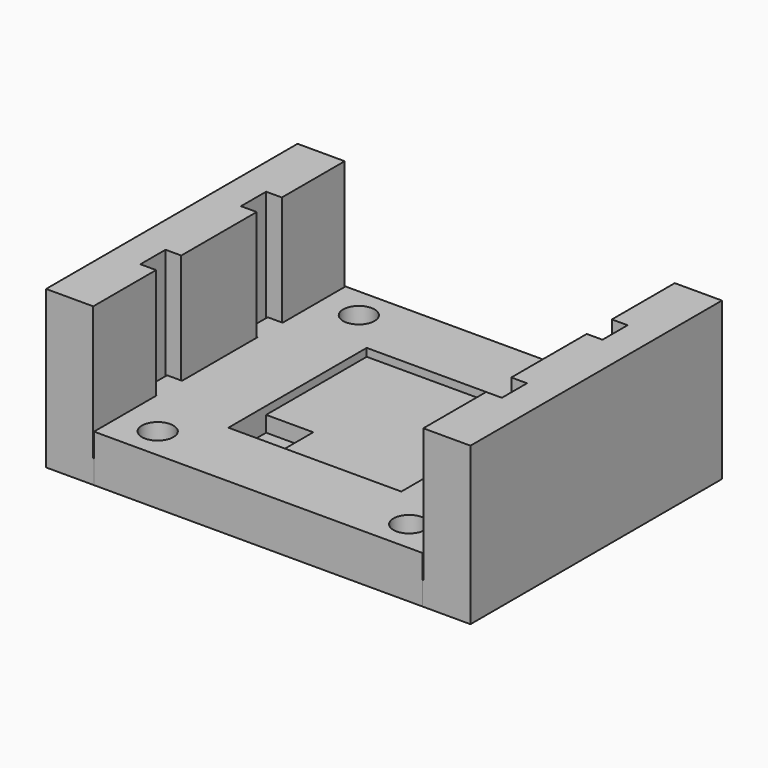
from build123d import *

# Parameters (mm, degrees)
F0_W      = 54
F0_H      = 40
F0_R      = 2
F0_R_2    = 3
F1_DEPTH  = 3
F3_DEPTH  = 20
F4_W      = 41.8
F4_H      = 40
F5_DEPTH  = 6
F7_START  = 5
F6_W      = 22
F6_H      = 22
F7_DEPTH  = 1
F9_START  = 2.5
F8_W      = 6
F8_H      = 6
F9_DEPTH  = 2.5
F12_R     = 2
F13_DEPTH = 25
F14_W     = 2
F14_H     = 4
F15_DEPTH = 6


# Not quite as in the source:
# - a feature of the source that left no trace in its solid (it failed there, or was rolled back) is left out


with BuildPart() as f1:
    # F0 (on Top) → F1 (new body)
    with BuildSketch(Plane.XY):
        Rectangle(F0_W, F0_H)
        with Locations((-16, -16)):
            Circle(F0_R, mode=Mode.SUBTRACT)
        with Locations((-4, -4)):
            Circle(F0_R_2, mode=Mode.SUBTRACT)
        with Locations((16, -16)):
            Circle(F0_R, mode=Mode.SUBTRACT)
        with Locations((4, -4)):
            Circle(F0_R_2, mode=Mode.SUBTRACT)
        with Locations((-4, 4)):
            Circle(F0_R_2, mode=Mode.SUBTRACT)
        with Locations((-16, 16)):
            Circle(F0_R, mode=Mode.SUBTRACT)
        with Locations((4, 4)):
            Circle(F0_R_2, mode=Mode.SUBTRACT)
        with Locations((16, 16)):
            Circle(F0_R, mode=Mode.SUBTRACT)
    extrude(amount=F1_DEPTH)

    # F2 (on Top) → F3 (join)
    with BuildSketch(Plane.XY):
        Polygon((-27, 12.5), (-27, -20), (-21, -20), (-21, -10), (-23, -10), (-23, -6), (-21, -6), (-21, 6), (-23, 6), (-23, 10), (-21, 10), (-21, 20), (-27, 20), align=None)
        Polygon((27, 20), (21, 20), (21, 10), (23, 10), (23, 6), (21, 6), (21, -6), (23, -6), (23, -10), (21, -10), (21, -20), (27, -20), align=None)
    extrude(amount=F3_DEPTH)


with BuildPart() as f5:
    # F4 (on Top) → F5 (new body)
    with BuildSketch(Plane.XY):
        Rectangle(F4_W, F4_H)
    extrude(amount=F5_DEPTH)

    # F6 (on Top) → F7 (cut)
    with BuildSketch(Plane.XY.offset(F7_START)):
        Rectangle(F6_W, F6_H)
    extrude(amount=F7_DEPTH, mode=Mode.SUBTRACT)

    # F8 (on Top) → F9 (cut)
    with BuildSketch(Plane.XY.offset(F9_START)):
        with Locations((-8, -8)):
            Rectangle(F8_W, F8_H)
    extrude(amount=F9_DEPTH, mode=Mode.SUBTRACT)

    # F12 (on Top) → F13 (cut)
    with BuildSketch(Plane.XY):
        with Locations((-16, 16)):
            Circle(F12_R)
        with Locations((16, 16)):
            Circle(F12_R)
        with Locations((16, -16)):
            Circle(F12_R)
        with Locations((-16, -16)):
            Circle(F12_R)
    extrude(amount=F13_DEPTH, mode=Mode.SUBTRACT)

    # F14 (on Top) → F15 (join)
    with BuildSketch(Plane.XY):
        with Locations((-21.8, 8)):
            Rectangle(F14_W, F14_H)
        with Locations((-21.8, -8)):
            Rectangle(F14_W, F14_H)
        with Locations((21.8, 8)):
            Rectangle(F14_W, F14_H)
        with Locations((21.8, -8)):
            Rectangle(F14_W, F14_H)
    extrude(amount=F15_DEPTH)


solid = Compound([f1.part, f5.part])
